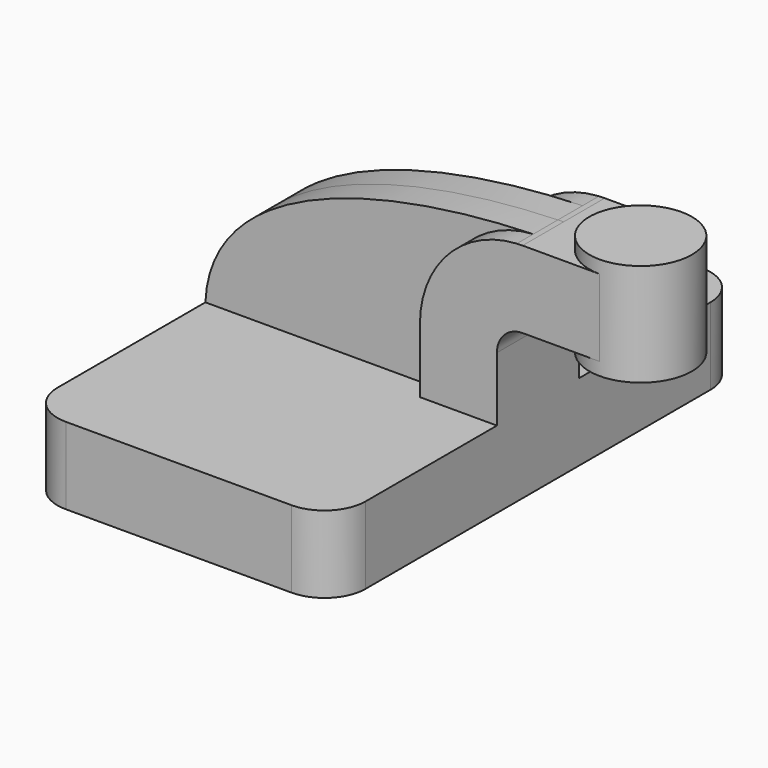
from build123d import *

# Parameters (mm, degrees)
F1_DEPTH = 63.5
F0_W     = 12.7
F0_H     = 19.05
F2_DEPTH = 12.7
F3_DEPTH = 7.62
F5_R     = 10.16


with BuildPart() as f1:
    # F0 (on Front) → F1 (new body, symmetric)
    with BuildSketch(Plane.XZ):
        Polygon((38.1, -9.525), (38.1, 9.525), (19.05, 9.525), (-38.1, 9.525), (-38.1, -9.525), align=None)
    extrude(amount=F1_DEPTH, both=True)

    # F0 (on Front) → F2 (join, symmetric)
    with BuildSketch(Plane.XZ):
        with BuildLine():
            Line((19.05, 9.525), (38.1, 9.525))
            Line((38.1, 9.525), (38.1, 25.4))
            ThreePointArc((38.1, 25.4), (39.9598719395, 29.8901280605), (44.45, 31.75))
            Line((44.45, 31.75), (50.8, 31.75))
            Line((50.8, 31.75), (50.8, 50.8))
            Line((50.8, 50.8), (44.45, 50.8))
            add(Edge.make_bspline(
                [(43.0234601168, 50.7599089896), (43.4990053985, 50.7747770293), (43.9745405837, 50.7881375185), (44.45, 50.8)],
                knots=[91.2068846399, 91.2068846399, 91.2068846399, 91.2068846399, 92.2937057713, 92.2937057713, 92.2937057713, 92.2937057713], degree=3))
            ThreePointArc((43.0234601168, 50.7599089896), (25.9920191647, 42.8488665386), (19.05, 25.4))
            Line((19.05, 25.4), (19.05, 9.525))
        make_face()
        with Locations((57.15, 41.275)):
            Rectangle(F0_W, F0_H)
    extrude(amount=F2_DEPTH, both=True)

    # F0 (on Front) → F3 (join, symmetric)
    with BuildSketch(Plane.XZ):
        with BuildLine():
            Line((-38.1, 9.525), (19.05, 9.525))
            Line((19.05, 9.525), (19.05, 25.4))
            ThreePointArc((19.05, 25.4), (25.9920191647, 42.8488665386), (43.0234601168, 50.7599089896))
            add(Edge.make_bspline(
                [(-38.1, 9.525), (-36.8639150117, 37.6472105963), (3.1153258394, 49.5121714006), (43.0234601168, 50.7599089896)],
                knots=[0, 0, 0, 0, 91.2068846399, 91.2068846399, 91.2068846399, 91.2068846399], degree=3))
        make_face()
    extrude(amount=F3_DEPTH, both=True)

    # F0 (on Front) → F4 (revolve)
    with BuildSketch(Plane.XZ):
        Polygon((63.5, 50.8), (63.5, 31.75), (63.5, 28.575), (76.2, 28.575), (76.2, 53.975), (63.5, 53.975), align=None)
    revolve(axis=Axis((63.5, 0, 41.275), (0, 0, 1)))

    # F5
    f5_edges = [f1.edges().sort_by_distance(p)[0] for p in [
        (38.1, -63.5, 0),
        (-38.1, -63.5, 0),
        (-38.1, 63.5, 0),
        (38.1, 63.5, 0),
    ]]
    fillet(f5_edges, radius=F5_R)


solid = f1.part
